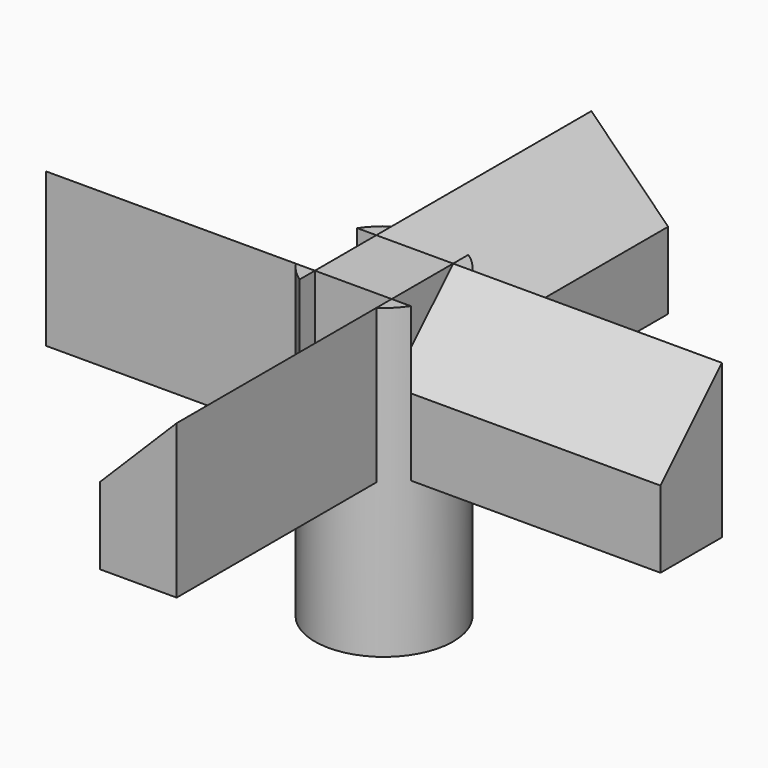
from build123d import *

# Parameters (mm, degrees)
F0_R     = 4.5
F1_DEPTH = 10
F2_W     = 5
F2_H     = 5
F3_DEPTH = 10
F4_SIZE  = 4.99999
F5_DEPTH = 10
F7_D     = 4
F7_DEPTH = 12
F7_TIP   = 1.2017212381


# Not quite as in the source:
# - a fillet or chamfer is up to 0.001 mm smaller than in the source, because OpenCascade refuses the exact size


with BuildPart() as f1:
    # F0 (on Top) → F1 (new body)
    with BuildSketch(Plane.XY):
        Circle(F0_R)
    extrude(amount=F1_DEPTH)

    # F2 (on face) → F3 (join)
    with BuildSketch(Plane.XY.offset(10)):
        with BuildLine():
            ThreePointArc((2.5, -3.7416573868), (0, -4.5), (-2.5, -3.7416573868))
            Line((-2.5, -3.7416573868), (-2.5, -20))
            Line((-2.5, -20), (2.5, -20))
            Line((2.5, -20), (2.5, -3.7416573868))
        make_face()
        with BuildLine():
            Line((-3.7416573868, 2.5), (-20, 2.5))
            Line((-20, 2.5), (-20, -2.5))
            Line((-20, -2.5), (-3.7416573868, -2.5))
            ThreePointArc((-3.7416573868, -2.5), (-4.5, 0), (-3.7416573868, 2.5))
        make_face()
        with BuildLine():
            Line((-2.5, 20), (-2.5, 3.7416573868))
            ThreePointArc((-2.5, 3.7416573868), (0, 4.5), (2.5, 3.7416573868))
            Line((2.5, 3.7416573868), (2.5, 20))
            Line((2.5, 20), (-2.5, 20))
        make_face()
        with BuildLine():
            Line((20, 2.5), (3.7416573868, 2.5))
            ThreePointArc((3.7416573868, 2.5), (4.3062430401, 1.3062430401), (4.5, 0))
            ThreePointArc((4.5, 0), (4.3062430401, -1.3062430401), (3.7416573868, -2.5))
            Line((3.7416573868, -2.5), (20, -2.5))
            Line((20, -2.5), (20, 2.5))
        make_face()
        with BuildLine():
            Line((3.7416573868, 2.5), (2.5, 2.5))
            Line((2.5, 2.5), (2.5, -2.5))
            Line((2.5, -2.5), (3.7416573868, -2.5))
            ThreePointArc((3.7416573868, -2.5), (4.3062430401, -1.3062430401), (4.5, 0))
            ThreePointArc((4.5, 0), (4.3062430401, 1.3062430401), (3.7416573868, 2.5))
        make_face()
        Rectangle(F2_W, F2_H)
        with BuildLine():
            Line((2.5, -2.5), (-2.5, -2.5))
            Line((-2.5, -2.5), (-2.5, -3.7416573868))
            ThreePointArc((-2.5, -3.7416573868), (0, -4.5), (2.5, -3.7416573868))
            Line((2.5, -3.7416573868), (2.5, -2.5))
        make_face()
        with BuildLine():
            Line((-2.5, 2.5), (-3.7416573868, 2.5))
            ThreePointArc((-3.7416573868, 2.5), (-4.5, 0), (-3.7416573868, -2.5))
            Line((-3.7416573868, -2.5), (-2.5, -2.5))
            Line((-2.5, -2.5), (-2.5, 2.5))
        make_face()
        with BuildLine():
            Line((-2.5, 3.7416573868), (-2.5, 2.5))
            Line((-2.5, 2.5), (2.5, 2.5))
            Line((2.5, 2.5), (2.5, 3.7416573868))
            ThreePointArc((2.5, 3.7416573868), (0, 4.5), (-2.5, 3.7416573868))
        make_face()
    extrude(amount=F3_DEPTH)

    # F4 (size 5 in the source; OpenCascade refuses exactly that, so slightly less here)
    f4_edges = [f1.edges().sort_by_distance(p)[0] for p in [
        (-2.5, -11.25, 20),
        (-11.25, 2.5, 20),
        (2.5, 11.25, 20),
        (11.25, -2.5, 20),
    ]]
    chamfer(f4_edges, length=F4_SIZE)

    # F5 (add): faces of the model
    f5_faces = [f1.faces().sort_by_distance(p)[0] for p in [
        (-2.940797231, 2.940797231, 10),
        (2.940797231, 2.940797231, 10),
        (2.940797231, -2.940797231, 10),
        (-2.940797231, -2.940797231, 10),
    ]]
    extrude(f5_faces, amount=F5_DEPTH)

    # F7
    with Locations(Plane(origin=(0, 0, 0), x_dir=(1, 0, 0), z_dir=(0, 0, -1))):
        with Locations((0, 0)):
            Hole(F7_D / 2, depth=F7_DEPTH)
            with Locations((0, 0, -(F7_DEPTH + F7_TIP / 2))):  # 118° drill point
                Cone(0, F7_D / 2, F7_TIP, mode=Mode.SUBTRACT)


solid = f1.part
